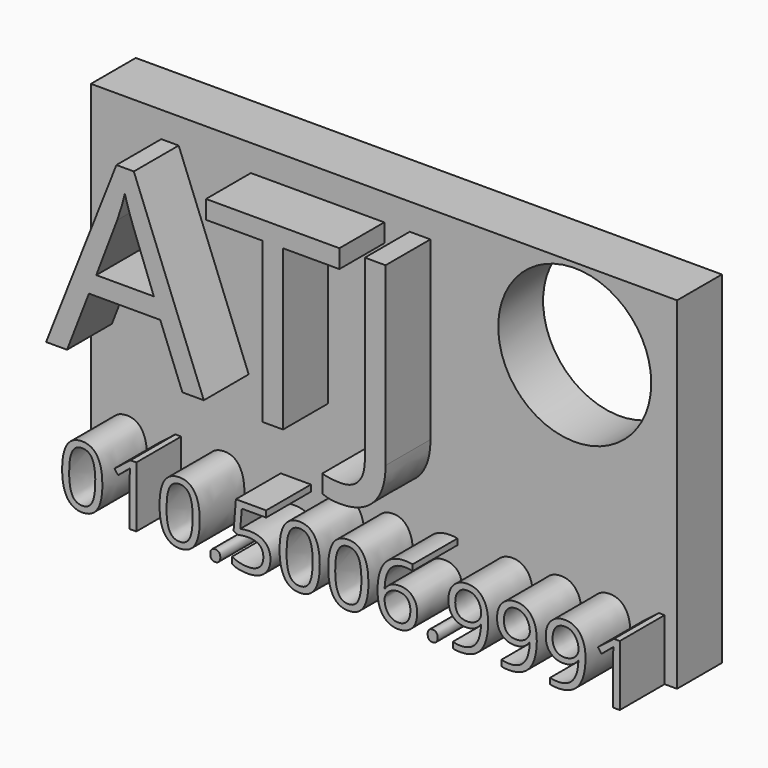
from build123d import *

# Parameters (mm, degrees)
F0_W         = 104.5464575291
F0_H         = 60.9978735447
F1_DEPTH     = 10
F2_TEXT_SIZE = 44.4611825246
F3_DEPTH     = 10
F4_TEXT_SIZE = 15.187646439
F5_DEPTH     = 10
F6_R         = 13.6458529722
F7_DEPTH     = 25.4


# Not quite as in the source:
# - Text() gives the source's letters only with a copy of the font that has no kerning and outlines rounded to 1/6400 em; it was checked with that copy


with BuildPart() as f1:
    # F0 (on Front) → F1 (new body)
    with BuildSketch(Plane.XZ):
        with Locations((52.2732287645, 30.4989367723)):
            Rectangle(F0_W, F0_H)
    extrude(amount=F1_DEPTH)

    # F2 (on face) → F3 (join)
    with BuildSketch(Plane.XZ.offset(10)):
        with Locations((0, 24.519553893)):
            Text('ATJ', F2_TEXT_SIZE, font='Open Sans', text_align=(TextAlign.LEFT, TextAlign.BOTTOM))
    extrude(amount=F3_DEPTH)

    # F4 (on face) → F5 (join)
    with BuildSketch(Plane.XZ.offset(10)):
        with Locations((2.1117358721, 0)):
            Text('010.5006.9991', F4_TEXT_SIZE, font='Open Sans', text_align=(TextAlign.LEFT, TextAlign.BOTTOM))
    extrude(amount=F5_DEPTH)

    # F6 (on face) → F7 (cut)
    with BuildSketch(Plane.XZ.offset(10)):
        with Locations((86.293309927, 46.4803464711)):
            Circle(F6_R)
    extrude(amount=-F7_DEPTH, mode=Mode.SUBTRACT)


solid = f1.part
